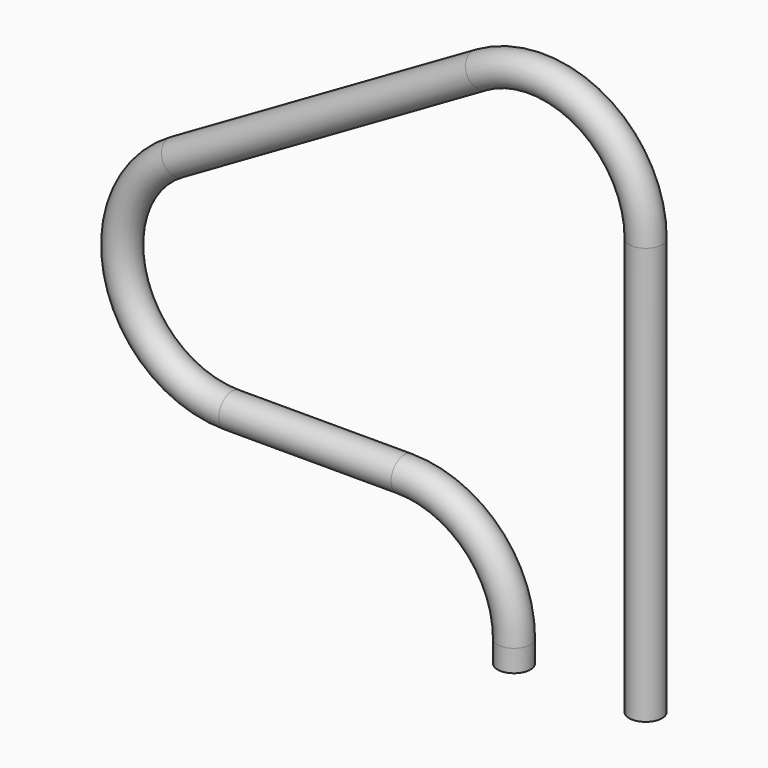
from build123d import *

# Parameters (mm, degrees)
F2_R   = 38.1
F2_R_2 = 25.4


with BuildPart() as f3:
    # F3: sweep along a path in F0
    with BuildLine(Plane.XZ) as f3_path:
        Line((0, 0), (0, 965.2))
        ThreePointArc((0, 965.2), (-127, 1185.1704525612), (-381, 1185.1704525612))
        Line((-381, 1185.1704525612), (-1084.905448196, 778.7704525612))
        ThreePointArc((-1084.905448196, 778.7704525612), (-1203.2506080734, 493.059962544), (-957.905448196, 304.8))
        Line((-957.905448196, 304.8), (-558.8, 304.8))
        ThreePointArc((-558.8, 304.8), (-379.1948775786, 230.4051224214), (-304.8, 50.8))
        Line((-304.8, 50.8), (-304.8, 0))
    # F2 (on line) → F3 (sweep)
    with BuildSketch(Plane.XY):
        Circle(F2_R)
        Circle(F2_R_2, mode=Mode.SUBTRACT)
    sweep(path=f3_path.line)


solid = f3.part
